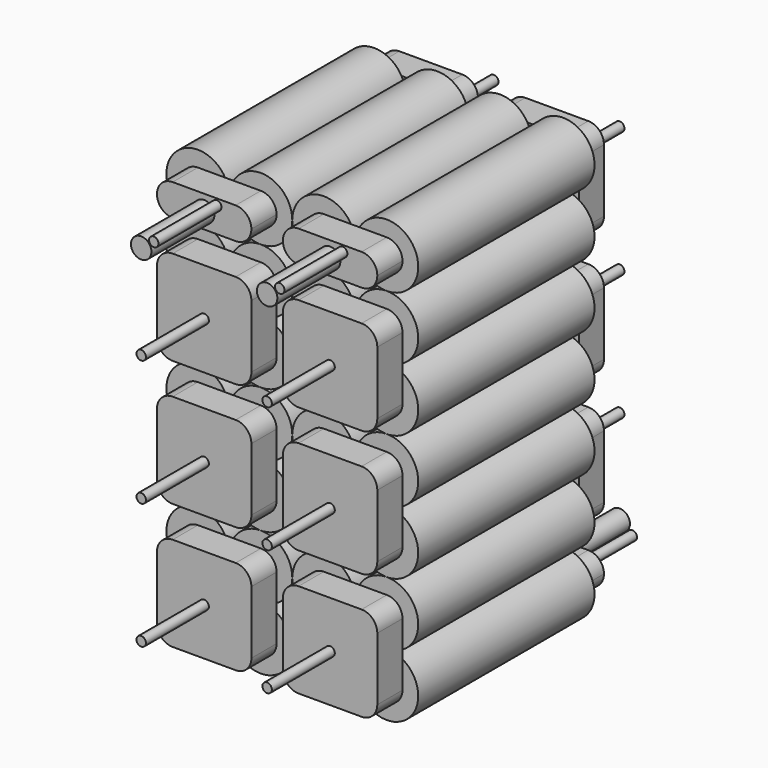
from build123d import *

# Parameters (mm, degrees)
F0_R      = 9.9995
F1_DEPTH  = 70
F2_W      = 30
F2_H      = 30
F3_DEPTH  = 10
F2_H_2    = 10
F4_W      = 30
F4_H      = 30
F5_DEPTH  = 10
F4_H_2    = 10
F6_R      = 4.99999
F6_2_R    = 4.99999
F6_3_R    = 4.99999
F6_4_R    = 4.99999
F6_5_R    = 4.99999
F6_6_R    = 4.99999
F6_7_R    = 4.99999
F6_8_R    = 4.99999
F6_9_R    = 4.99999
F6_10_R   = 4.99999
F6_11_R   = 4.99999
F6_12_R   = 4.99999
F6_13_R   = 4.99999
F6_14_R   = 4.99999
F6_15_R   = 4.99999
F6_16_R   = 4.99999
F7_R      = 1.5
F8_DEPTH  = 25
F7_R_2    = 3.25
F9_R      = 3.25
F10_DEPTH = 25
F9_R_2    = 1.5


# Not quite as in the source:
# - a fillet or chamfer is up to 0.001 mm smaller than in the source, because OpenCascade refuses the exact size


with BuildPart() as f1:
    # F0 (on Front) → F1 (new body)
    with BuildSketch(Plane.XZ):
        with Locations((10, 10)):
            Circle(F0_R)
    extrude(amount=F1_DEPTH)


with BuildPart() as f1b:
    # F0 (on Front) → F1, piece 2 (new body)
    with BuildSketch(Plane.XZ):
        with Locations((30, 10)):
            Circle(F0_R)
    extrude(amount=F1_DEPTH)


with BuildPart() as f1c:
    # F0 (on Front) → F1, piece 3 (new body)
    with BuildSketch(Plane.XZ):
        with Locations((50, 10)):
            Circle(F0_R)
    extrude(amount=F1_DEPTH)


with BuildPart() as f1d:
    # F0 (on Front) → F1, piece 4 (new body)
    with BuildSketch(Plane.XZ):
        with Locations((70, 10)):
            Circle(F0_R)
    extrude(amount=F1_DEPTH)


with BuildPart() as f1e:
    # F0 (on Front) → F1, piece 5 (new body)
    with BuildSketch(Plane.XZ):
        with Locations((10, 30)):
            Circle(F0_R)
    extrude(amount=F1_DEPTH)


with BuildPart() as f1f:
    # F0 (on Front) → F1, piece 6 (new body)
    with BuildSketch(Plane.XZ):
        with Locations((30, 30)):
            Circle(F0_R)
    extrude(amount=F1_DEPTH)


with BuildPart() as f1g:
    # F0 (on Front) → F1, piece 7 (new body)
    with BuildSketch(Plane.XZ):
        with Locations((50, 30)):
            Circle(F0_R)
    extrude(amount=F1_DEPTH)


with BuildPart() as f1h:
    # F0 (on Front) → F1, piece 8 (new body)
    with BuildSketch(Plane.XZ):
        with Locations((70, 30)):
            Circle(F0_R)
    extrude(amount=F1_DEPTH)


with BuildPart() as f1i:
    # F0 (on Front) → F1, piece 9 (new body)
    with BuildSketch(Plane.XZ):
        with Locations((10, 50)):
            Circle(F0_R)
    extrude(amount=F1_DEPTH)


with BuildPart() as f1j:
    # F0 (on Front) → F1, piece 10 (new body)
    with BuildSketch(Plane.XZ):
        with Locations((30, 50)):
            Circle(F0_R)
    extrude(amount=F1_DEPTH)


with BuildPart() as f1k:
    # F0 (on Front) → F1, piece 11 (new body)
    with BuildSketch(Plane.XZ):
        with Locations((50, 50)):
            Circle(F0_R)
    extrude(amount=F1_DEPTH)


with BuildPart() as f1l:
    # F0 (on Front) → F1, piece 12 (new body)
    with BuildSketch(Plane.XZ):
        with Locations((70, 50)):
            Circle(F0_R)
    extrude(amount=F1_DEPTH)


with BuildPart() as f1m:
    # F0 (on Front) → F1, piece 13 (new body)
    with BuildSketch(Plane.XZ):
        with Locations((10, 70)):
            Circle(F0_R)
    extrude(amount=F1_DEPTH)


with BuildPart() as f1n:
    # F0 (on Front) → F1, piece 14 (new body)
    with BuildSketch(Plane.XZ):
        with Locations((30, 70)):
            Circle(F0_R)
    extrude(amount=F1_DEPTH)


with BuildPart() as f1o:
    # F0 (on Front) → F1, piece 15 (new body)
    with BuildSketch(Plane.XZ):
        with Locations((50, 70)):
            Circle(F0_R)
    extrude(amount=F1_DEPTH)


with BuildPart() as f1p:
    # F0 (on Front) → F1, piece 16 (new body)
    with BuildSketch(Plane.XZ):
        with Locations((70, 70)):
            Circle(F0_R)
    extrude(amount=F1_DEPTH)


with BuildPart() as f1q:
    # F0 (on Front) → F1, piece 17 (new body)
    with BuildSketch(Plane.XZ):
        with Locations((10, 90)):
            Circle(F0_R)
    extrude(amount=F1_DEPTH)


with BuildPart() as f1r:
    # F0 (on Front) → F1, piece 18 (new body)
    with BuildSketch(Plane.XZ):
        with Locations((30, 90)):
            Circle(F0_R)
    extrude(amount=F1_DEPTH)


with BuildPart() as f1s:
    # F0 (on Front) → F1, piece 19 (new body)
    with BuildSketch(Plane.XZ):
        with Locations((50, 90)):
            Circle(F0_R)
    extrude(amount=F1_DEPTH)


with BuildPart() as f1t:
    # F0 (on Front) → F1, piece 20 (new body)
    with BuildSketch(Plane.XZ):
        with Locations((70, 90)):
            Circle(F0_R)
    extrude(amount=F1_DEPTH)


with BuildPart() as f1u:
    # F0 (on Front) → F1, piece 21 (new body)
    with BuildSketch(Plane.XZ):
        with Locations((10, 110)):
            Circle(F0_R)
    extrude(amount=F1_DEPTH)


with BuildPart() as f1v:
    # F0 (on Front) → F1, piece 22 (new body)
    with BuildSketch(Plane.XZ):
        with Locations((30, 110)):
            Circle(F0_R)
    extrude(amount=F1_DEPTH)


with BuildPart() as f1w:
    # F0 (on Front) → F1, piece 23 (new body)
    with BuildSketch(Plane.XZ):
        with Locations((50, 110)):
            Circle(F0_R)
    extrude(amount=F1_DEPTH)


with BuildPart() as f1x:
    # F0 (on Front) → F1, piece 24 (new body)
    with BuildSketch(Plane.XZ):
        with Locations((70, 110)):
            Circle(F0_R)
    extrude(amount=F1_DEPTH)


with BuildPart() as f1y:
    # F0 (on Front) → F1, piece 25 (new body)
    with BuildSketch(Plane.XZ):
        with Locations((10, 130)):
            Circle(F0_R)
    extrude(amount=F1_DEPTH)


with BuildPart() as f1z:
    # F0 (on Front) → F1, piece 26 (new body)
    with BuildSketch(Plane.XZ):
        with Locations((30, 130)):
            Circle(F0_R)
    extrude(amount=F1_DEPTH)


with BuildPart() as f1ba:
    # F0 (on Front) → F1, piece 27 (new body)
    with BuildSketch(Plane.XZ):
        with Locations((50, 130)):
            Circle(F0_R)
    extrude(amount=F1_DEPTH)


with BuildPart() as f1bb:
    # F0 (on Front) → F1, piece 28 (new body)
    with BuildSketch(Plane.XZ):
        with Locations((70, 130)):
            Circle(F0_R)
    extrude(amount=F1_DEPTH)


with BuildPart() as f3:
    # F2 (on face) → F3 (new body)
    with BuildSketch(Plane.XZ.offset(70)):
        with Locations((20, 20)):
            Rectangle(F2_W, F2_H)
    extrude(amount=F3_DEPTH)

    # F6#7 (radius 5 in the source; OpenCascade refuses exactly that, so slightly less here)
    f6_7_edges = [f3.edges().sort_by_distance(p)[0] for p in [
        (5, -75, 35),
        (35, -75, 35),
        (35, -75, 5),
        (5, -75, 5),
    ]]
    fillet(f6_7_edges, radius=F6_7_R)


with BuildPart() as f3b:
    # F2 (on face) → F3, piece 2 (new body)
    with BuildSketch(Plane.XZ.offset(70)):
        with Locations((60, 20)):
            Rectangle(F2_W, F2_H)
    extrude(amount=F3_DEPTH)

    # F6#8 (radius 5 in the source; OpenCascade refuses exactly that, so slightly less here)
    f6_8_edges = [f3b.edges().sort_by_distance(p)[0] for p in [
        (45, -75, 35),
        (75, -75, 35),
        (75, -75, 5),
        (45, -75, 5),
    ]]
    fillet(f6_8_edges, radius=F6_8_R)


with BuildPart() as f3c:
    # F2 (on face) → F3, piece 3 (new body)
    with BuildSketch(Plane.XZ.offset(70)):
        with Locations((20, 60)):
            Rectangle(F2_W, F2_H)
    extrude(amount=F3_DEPTH)

    # F6#5 (radius 5 in the source; OpenCascade refuses exactly that, so slightly less here)
    f6_5_edges = [f3c.edges().sort_by_distance(p)[0] for p in [
        (5, -75, 75),
        (35, -75, 75),
        (35, -75, 45),
        (5, -75, 45),
    ]]
    fillet(f6_5_edges, radius=F6_5_R)


with BuildPart() as f3d:
    # F2 (on face) → F3, piece 4 (new body)
    with BuildSketch(Plane.XZ.offset(70)):
        with Locations((60, 60)):
            Rectangle(F2_W, F2_H)
    extrude(amount=F3_DEPTH)

    # F6#6 (radius 5 in the source; OpenCascade refuses exactly that, so slightly less here)
    f6_6_edges = [f3d.edges().sort_by_distance(p)[0] for p in [
        (45, -75, 75),
        (75, -75, 75),
        (75, -75, 45),
        (45, -75, 45),
    ]]
    fillet(f6_6_edges, radius=F6_6_R)


with BuildPart() as f3e:
    # F2 (on face) → F3, piece 5 (new body)
    with BuildSketch(Plane.XZ.offset(70)):
        with Locations((20, 100)):
            Rectangle(F2_W, F2_H)
    extrude(amount=F3_DEPTH)

    # F6#4 (radius 5 in the source; OpenCascade refuses exactly that, so slightly less here)
    f6_4_edges = [f3e.edges().sort_by_distance(p)[0] for p in [
        (5, -75, 115),
        (35, -75, 115),
        (35, -75, 85),
        (5, -75, 85),
    ]]
    fillet(f6_4_edges, radius=F6_4_R)


with BuildPart() as f3f:
    # F2 (on face) → F3, piece 6 (new body)
    with BuildSketch(Plane.XZ.offset(70)):
        with Locations((60, 100)):
            Rectangle(F2_W, F2_H)
    extrude(amount=F3_DEPTH)

    # F6#2 (radius 5 in the source; OpenCascade refuses exactly that, so slightly less here)
    f6_2_edges = [f3f.edges().sort_by_distance(p)[0] for p in [
        (75, -75, 115),
        (75, -75, 85),
        (45, -75, 115),
        (45, -75, 85),
    ]]
    fillet(f6_2_edges, radius=F6_2_R)


with BuildPart() as f3g:
    # F2 (on face) → F3, piece 7 (new body)
    with BuildSketch(Plane.XZ.offset(70)):
        with Locations((20, 130)):
            Rectangle(F2_W, F2_H_2)
    extrude(amount=F3_DEPTH)

    # F6#3 (radius 5 in the source; OpenCascade refuses exactly that, so slightly less here)
    f6_3_edges = [f3g.edges().sort_by_distance(p)[0] for p in [
        (35, -75, 135),
        (5, -75, 135),
        (35, -75, 125),
        (5, -75, 125),
    ]]
    fillet(f6_3_edges, radius=F6_3_R)


with BuildPart() as f3h:
    # F2 (on face) → F3, piece 8 (new body)
    with BuildSketch(Plane.XZ.offset(70)):
        with Locations((60, 130)):
            Rectangle(F2_W, F2_H_2)
    extrude(amount=F3_DEPTH)

    # F6 (radius 5 in the source; OpenCascade refuses exactly that, so slightly less here)
    f6_edges = [f3h.edges().sort_by_distance(p)[0] for p in [
        (75, -75, 135),
        (75, -75, 125),
        (45, -75, 135),
        (45, -75, 125),
    ]]
    fillet(f6_edges, radius=F6_R)


with BuildPart() as f5:
    # F4 (on face) → F5 (new body)
    with BuildSketch(Plane(origin=(0, 0, 0), x_dir=(-1, 0, 0), z_dir=(0, 1, 0))):
        with Locations((-60, 40)):
            Rectangle(F4_W, F4_H)
    extrude(amount=F5_DEPTH)

    # F6#12 (radius 5 in the source; OpenCascade refuses exactly that, so slightly less here)
    f6_12_edges = [f5.edges().sort_by_distance(p)[0] for p in [
        (45, 5, 25),
        (75, 5, 25),
        (45, 5, 55),
        (75, 5, 55),
    ]]
    fillet(f6_12_edges, radius=F6_12_R)


with BuildPart() as f5b:
    # F4 (on face) → F5, piece 2 (new body)
    with BuildSketch(Plane(origin=(0, 0, 0), x_dir=(-1, 0, 0), z_dir=(0, 1, 0))):
        with Locations((-20, 40)):
            Rectangle(F4_W, F4_H)
    extrude(amount=F5_DEPTH)

    # F6#10 (radius 5 in the source; OpenCascade refuses exactly that, so slightly less here)
    f6_10_edges = [f5b.edges().sort_by_distance(p)[0] for p in [
        (5, 5, 25),
        (35, 5, 25),
        (5, 5, 55),
        (35, 5, 55),
    ]]
    fillet(f6_10_edges, radius=F6_10_R)


with BuildPart() as f5c:
    # F4 (on face) → F5, piece 3 (new body)
    with BuildSketch(Plane(origin=(0, 0, 0), x_dir=(-1, 0, 0), z_dir=(0, 1, 0))):
        with Locations((-60, 80)):
            Rectangle(F4_W, F4_H)
    extrude(amount=F5_DEPTH)

    # F6#13 (radius 5 in the source; OpenCascade refuses exactly that, so slightly less here)
    f6_13_edges = [f5c.edges().sort_by_distance(p)[0] for p in [
        (75, 5, 65),
        (45, 5, 65),
        (45, 5, 95),
        (75, 5, 95),
    ]]
    fillet(f6_13_edges, radius=F6_13_R)


with BuildPart() as f5d:
    # F4 (on face) → F5, piece 4 (new body)
    with BuildSketch(Plane(origin=(0, 0, 0), x_dir=(-1, 0, 0), z_dir=(0, 1, 0))):
        with Locations((-20, 80)):
            Rectangle(F4_W, F4_H)
    extrude(amount=F5_DEPTH)

    # F6#14 (radius 5 in the source; OpenCascade refuses exactly that, so slightly less here)
    f6_14_edges = [f5d.edges().sort_by_distance(p)[0] for p in [
        (35, 5, 65),
        (5, 5, 65),
        (5, 5, 95),
        (35, 5, 95),
    ]]
    fillet(f6_14_edges, radius=F6_14_R)


with BuildPart() as f5e:
    # F4 (on face) → F5, piece 5 (new body)
    with BuildSketch(Plane(origin=(0, 0, 0), x_dir=(-1, 0, 0), z_dir=(0, 1, 0))):
        with Locations((-60, 120)):
            Rectangle(F4_W, F4_H)
    extrude(amount=F5_DEPTH)

    # F6#16 (radius 5 in the source; OpenCascade refuses exactly that, so slightly less here)
    f6_16_edges = [f5e.edges().sort_by_distance(p)[0] for p in [
        (45, 5, 105),
        (75, 5, 105),
        (45, 5, 135),
        (75, 5, 135),
    ]]
    fillet(f6_16_edges, radius=F6_16_R)


with BuildPart() as f5f:
    # F4 (on face) → F5, piece 6 (new body)
    with BuildSketch(Plane(origin=(0, 0, 0), x_dir=(-1, 0, 0), z_dir=(0, 1, 0))):
        with Locations((-20, 120)):
            Rectangle(F4_W, F4_H)
    extrude(amount=F5_DEPTH)

    # F6#15 (radius 5 in the source; OpenCascade refuses exactly that, so slightly less here)
    f6_15_edges = [f5f.edges().sort_by_distance(p)[0] for p in [
        (5, 5, 105),
        (35, 5, 105),
        (5, 5, 135),
        (35, 5, 135),
    ]]
    fillet(f6_15_edges, radius=F6_15_R)


with BuildPart() as f5g:
    # F4 (on face) → F5, piece 7 (new body)
    with BuildSketch(Plane(origin=(0, 0, 0), x_dir=(-1, 0, 0), z_dir=(0, 1, 0))):
        with Locations((-60, 10)):
            Rectangle(F4_W, F4_H_2)
    extrude(amount=F5_DEPTH)

    # F6#11 (radius 5 in the source; OpenCascade refuses exactly that, so slightly less here)
    f6_11_edges = [f5g.edges().sort_by_distance(p)[0] for p in [
        (45, 5, 5),
        (45, 5, 15),
        (75, 5, 5),
        (75, 5, 15),
    ]]
    fillet(f6_11_edges, radius=F6_11_R)


with BuildPart() as f5h:
    # F4 (on face) → F5, piece 8 (new body)
    with BuildSketch(Plane(origin=(0, 0, 0), x_dir=(-1, 0, 0), z_dir=(0, 1, 0))):
        with Locations((-20, 10)):
            Rectangle(F4_W, F4_H_2)
    extrude(amount=F5_DEPTH)

    # F6#9 (radius 5 in the source; OpenCascade refuses exactly that, so slightly less here)
    f6_9_edges = [f5h.edges().sort_by_distance(p)[0] for p in [
        (5, 5, 5),
        (35, 5, 5),
        (5, 5, 15),
        (35, 5, 15),
    ]]
    fillet(f6_9_edges, radius=F6_9_R)


with BuildPart() as f8:
    # F7 (on face) → F8 (new body)
    with BuildSketch(Plane(origin=(0, 10, 0), x_dir=(-1, 0, 0), z_dir=(0, 1, 0))):
        with Locations((-60, 120)):
            Circle(F7_R)
    extrude(amount=F8_DEPTH)


with BuildPart() as f8b:
    # F7 (on face) → F8, piece 2 (new body)
    with BuildSketch(Plane(origin=(0, 10, 0), x_dir=(-1, 0, 0), z_dir=(0, 1, 0))):
        with Locations((-20, 120)):
            Circle(F7_R)
    extrude(amount=F8_DEPTH)


with BuildPart() as f8c:
    # F7 (on face) → F8, piece 3 (new body)
    with BuildSketch(Plane(origin=(0, 10, 0), x_dir=(-1, 0, 0), z_dir=(0, 1, 0))):
        with Locations((-60, 80)):
            Circle(F7_R)
    extrude(amount=F8_DEPTH)


with BuildPart() as f8d:
    # F7 (on face) → F8, piece 4 (new body)
    with BuildSketch(Plane(origin=(0, 10, 0), x_dir=(-1, 0, 0), z_dir=(0, 1, 0))):
        with Locations((-20, 80)):
            Circle(F7_R)
    extrude(amount=F8_DEPTH)


with BuildPart() as f8e:
    # F7 (on face) → F8, piece 5 (new body)
    with BuildSketch(Plane(origin=(0, 10, 0), x_dir=(-1, 0, 0), z_dir=(0, 1, 0))):
        with Locations((-60, 40)):
            Circle(F7_R)
    extrude(amount=F8_DEPTH)


with BuildPart() as f8f:
    # F7 (on face) → F8, piece 6 (new body)
    with BuildSketch(Plane(origin=(0, 10, 0), x_dir=(-1, 0, 0), z_dir=(0, 1, 0))):
        with Locations((-20, 40)):
            Circle(F7_R)
    extrude(amount=F8_DEPTH)


with BuildPart() as f8g:
    # F7 (on face) → F8, piece 7 (new body)
    with BuildSketch(Plane(origin=(0, 10, 0), x_dir=(-1, 0, 0), z_dir=(0, 1, 0))):
        with Locations((-60, 10)):
            Circle(F7_R_2)
    extrude(amount=F8_DEPTH)


with BuildPart() as f8h:
    # F7 (on face) → F8, piece 8 (new body)
    with BuildSketch(Plane(origin=(0, 10, 0), x_dir=(-1, 0, 0), z_dir=(0, 1, 0))):
        with Locations((-20, 10)):
            Circle(F7_R_2)
    extrude(amount=F8_DEPTH)


with BuildPart() as f8i:
    # F7 (on face) → F8, piece 9 (new body)
    with BuildSketch(Plane(origin=(0, 10, 0), x_dir=(-1, 0, 0), z_dir=(0, 1, 0))):
        with Locations((-64, 7)):
            Circle(F7_R)
    extrude(amount=F8_DEPTH)


with BuildPart() as f8j:
    # F7 (on face) → F8, piece 10 (new body)
    with BuildSketch(Plane(origin=(0, 10, 0), x_dir=(-1, 0, 0), z_dir=(0, 1, 0))):
        with Locations((-24, 7)):
            Circle(F7_R)
    extrude(amount=F8_DEPTH)


with BuildPart() as f10:
    # F9 (on face) → F10 (new body)
    with BuildSketch(Plane.XZ.offset(80)):
        with Locations((20, 130)):
            Circle(F9_R)
    extrude(amount=F10_DEPTH)


with BuildPart() as f10b:
    # F9 (on face) → F10, piece 2 (new body)
    with BuildSketch(Plane.XZ.offset(80)):
        with Locations((60, 130)):
            Circle(F9_R)
    extrude(amount=F10_DEPTH)


with BuildPart() as f10c:
    # F9 (on face) → F10, piece 3 (new body)
    with BuildSketch(Plane.XZ.offset(80)):
        with Locations((20, 100)):
            Circle(F9_R_2)
    extrude(amount=F10_DEPTH)


with BuildPart() as f10d:
    # F9 (on face) → F10, piece 4 (new body)
    with BuildSketch(Plane.XZ.offset(80)):
        with Locations((60, 100)):
            Circle(F9_R_2)
    extrude(amount=F10_DEPTH)


with BuildPart() as f10e:
    # F9 (on face) → F10, piece 5 (new body)
    with BuildSketch(Plane.XZ.offset(80)):
        with Locations((20, 60)):
            Circle(F9_R_2)
    extrude(amount=F10_DEPTH)


with BuildPart() as f10f:
    # F9 (on face) → F10, piece 6 (new body)
    with BuildSketch(Plane.XZ.offset(80)):
        with Locations((60, 60)):
            Circle(F9_R_2)
    extrude(amount=F10_DEPTH)


with BuildPart() as f10g:
    # F9 (on face) → F10, piece 7 (new body)
    with BuildSketch(Plane.XZ.offset(80)):
        with Locations((20, 20)):
            Circle(F9_R_2)
    extrude(amount=F10_DEPTH)


with BuildPart() as f10h:
    # F9 (on face) → F10, piece 8 (new body)
    with BuildSketch(Plane.XZ.offset(80)):
        with Locations((60, 20)):
            Circle(F9_R_2)
    extrude(amount=F10_DEPTH)


with BuildPart() as f10i:
    # F9 (on face) → F10, piece 9 (new body)
    with BuildSketch(Plane.XZ.offset(80)):
        with Locations((24, 133)):
            Circle(F9_R_2)
    extrude(amount=F10_DEPTH)


with BuildPart() as f10j:
    # F9 (on face) → F10, piece 10 (new body)
    with BuildSketch(Plane.XZ.offset(80)):
        with Locations((64, 133)):
            Circle(F9_R_2)
    extrude(amount=F10_DEPTH)


solid = Compound([f1.part, f1b.part, f1c.part, f1d.part, f1e.part, f1f.part, f1g.part, f1h.part, f1i.part, f1j.part, f1k.part, f1l.part, f1m.part, f1n.part, f1o.part, f1p.part, f1q.part, f1r.part, f1s.part, f1t.part, f1u.part, f1v.part, f1w.part, f1x.part, f1y.part, f1z.part, f1ba.part, f1bb.part, f3.part, f3b.part, f3c.part, f3d.part, f3e.part, f3f.part, f3g.part, f3h.part, f5.part, f5b.part, f5c.part, f5d.part, f5e.part, f5f.part, f5g.part, f5h.part, f8.part, f8b.part, f8c.part, f8d.part, f8e.part, f8f.part, f8g.part, f8h.part, f8i.part, f8j.part, f10.part, f10b.part, f10c.part, f10d.part, f10e.part, f10f.part, f10g.part, f10h.part, f10i.part, f10j.part])
